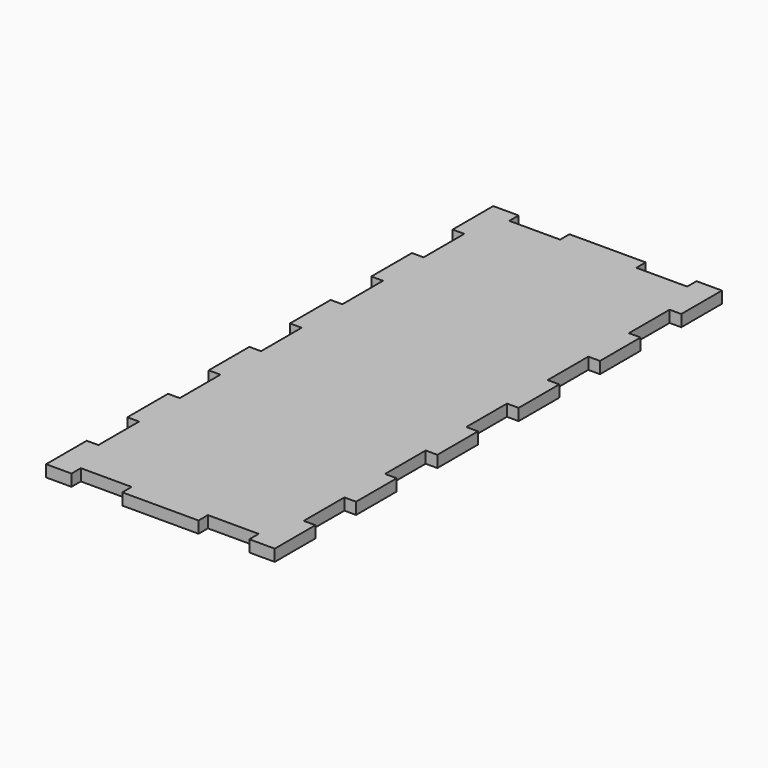
from build123d import *

# Parameters (mm, degrees)
F0_W     = 114.3
F0_H     = 279.4
F1_DEPTH = 5.842
F2_W     = 5.842
F2_H     = 25.4
F2_W_2   = 25.4
F2_H_2   = 5.842
F3_DEPTH = 5.842


# Not quite as in the source:
# - a feature names something its author has since deleted; it is built from what else it names


with BuildPart() as f1:
    # F0 (on Top) → F1 (new body)
    with BuildSketch(Plane.XY):
        with Locations((-3.3015739173, 43.0149683578)):
            Rectangle(F0_W, F0_H)
    extrude(amount=F1_DEPTH)

    # F2 (on face) → F3 (cut, through all)
    with BuildSketch(Plane.XY.offset(5.842)):
        with Locations((50.9274260827, 93.8149683578)):
            Rectangle(F2_W, F2_H)
        with Locations((-57.5305739173, 93.8149683578)):
            Rectangle(F2_W, F2_H)
        with Locations((-57.5305739173, 43.0149683578)):
            Rectangle(F2_W, F2_H)
        with Locations((50.9274260827, 43.0149683578)):
            Rectangle(F2_W, F2_H)
        with Locations((50.9274260827, -7.7850316422)):
            Rectangle(F2_W, F2_H)
        with Locations((50.9274260827, -58.5850316422)):
            Rectangle(F2_W, F2_H)
        with Locations((28.4484260827, -93.7640316422)):
            Rectangle(F2_W_2, F2_H_2)
        with Locations((-35.0515739173, -93.7640316422)):
            Rectangle(F2_W_2, F2_H_2)
        with Locations((-57.5305739173, -58.5850316422)):
            Rectangle(F2_W, F2_H)
        with Locations((-57.5305739173, -7.7850316422)):
            Rectangle(F2_W, F2_H)
        with Locations((28.4484260827, 179.7939683578)):
            Rectangle(F2_W_2, F2_H_2)
        with Locations((-35.0515739173, 179.7939683578)):
            Rectangle(F2_W_2, F2_H_2)
        with Locations((-57.5305739173, 144.6149683578)):
            Rectangle(F2_W, F2_H)
        with Locations((50.9274260827, 144.6149683578)):
            Rectangle(F2_W, F2_H)
    extrude(amount=-F3_DEPTH, mode=Mode.SUBTRACT)


solid = f1.part
